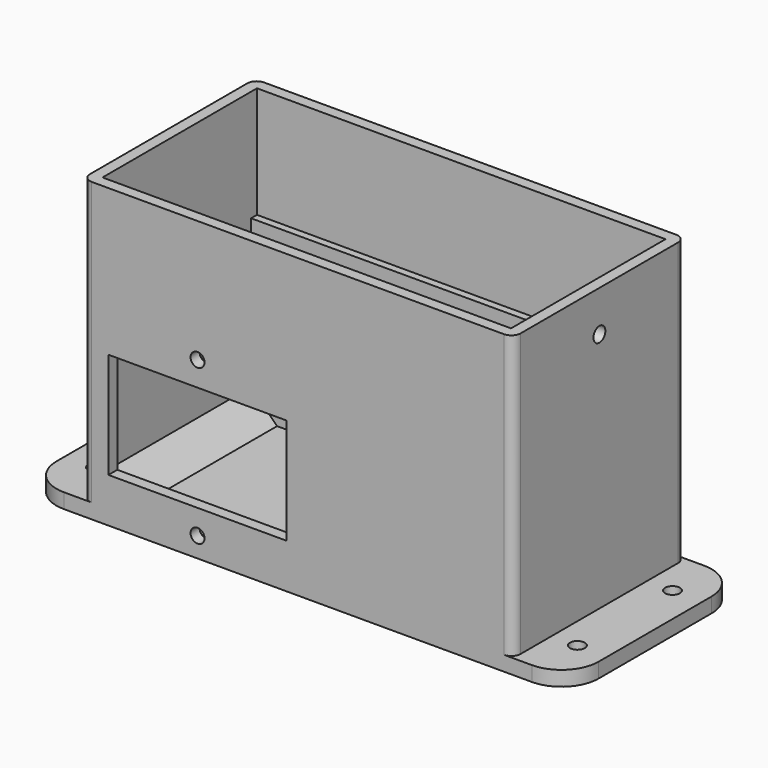
from build123d import *

# Parameters (mm, degrees)
F0_W      = 116
F0_H      = 58
F1_DEPTH  = 80
F2_T      = -3
F4_DEPTH  = 47
F5_R      = 2
F6_DEPTH  = 3.001
F7_W      = 58
F7_H      = 4
F8_DEPTH  = 15
F9_R      = 10
F10_R     = 2
F11_DEPTH = 4.001
F12_W     = 48
F12_H     = 28.5
F13_DEPTH = 5
F14_R     = 1.875
F15_DEPTH = 5
F16_W     = 25
F16_H     = 5
F17_DEPTH = 5.001
F18_R     = 2.49999
F19_R     = 2.5
F20_SIZE  = 7


# Not quite as in the source:
# - a fillet or chamfer is up to 0.001 mm smaller than in the source, because OpenCascade refuses the exact size
# - a pattern or mirror of a feature is missing from the dataset's text; its kind, count and spacing are read off the source's solid


with BuildPart() as f1:
    # F0 (on Top) → F1 (new body)
    with BuildSketch(Plane.XY):
        Rectangle(F0_W, F0_H)
    extrude(amount=F1_DEPTH)

    # F2
    f2_openings = [f1.faces().sort_by_distance(p)[0] for p in [
        (0, 0, 80),
    ]]
    offset(amount=F2_T, openings=f2_openings)

    # F3 (on face) → F4 (join)
    with BuildSketch(Plane.XY.offset(3)):
        Polygon((-55, 26), (-55, 24), (53, 24), (53, -26), (55, -26), (55, 26), align=None)
    extrude(amount=F4_DEPTH)

    # F5 (on face) → F6 (cut, through all)
    with BuildSketch(Plane(origin=(55, 0, 0), x_dir=(0, -1, 0), z_dir=(-1, 0, 0))):
        with Locations((0, 69)):
            Circle(F5_R)
    extrude(amount=-F6_DEPTH, mode=Mode.SUBTRACT)

    # F7 (on face) → F8 (join)
    with BuildSketch(Plane.YZ.offset(58)):
        with Locations((0, 2)):
            Rectangle(F7_W, F7_H)
    f8 = extrude(amount=F8_DEPTH)

    # F8_copies: F8 across plane
    add(f8.mirror(Plane(origin=(0, 0, 0), x_dir=(0, 0, -1), z_dir=(-1, 0, 0))))

    # F9
    f9_edges = [f1.edges().sort_by_distance(p)[0] for p in [
        (73, 29, 2),
        (73, -29, 2),
        (-73, -29, 2),
        (-73, 29, 2),
    ]]
    fillet(f9_edges, radius=F9_R)

    # F10 (on face) → F11 (cut, through all)
    with BuildSketch(Plane.XY.offset(4)):
        with Locations((64.8827031255, 16)):
            Circle(F10_R)
        with Locations((64.8827031255, -16)):
            Circle(F10_R)
    f11 = extrude(amount=-F11_DEPTH, mode=Mode.SUBTRACT)

    # F11_copies: F11 across plane
    add(f11.mirror(Plane(origin=(0, 0, 0), x_dir=(0, 0, -1), z_dir=(-1, 0, 0))), mode=Mode.SUBTRACT)

    # F12 (on face) → F13 (cut)
    with BuildSketch(Plane.XZ.offset(29)):
        with Locations((-27, 26.25)):
            Rectangle(F12_W, F12_H)
    extrude(amount=-F13_DEPTH, mode=Mode.SUBTRACT)

    # F14 (on face) → F15 (cut)
    with BuildSketch(Plane.XZ.offset(29)):
        with Locations((-27, 47.1)):
            Circle(F14_R)
        with Locations((-27, 5.4)):
            Circle(F14_R)
    extrude(amount=-F15_DEPTH, mode=Mode.SUBTRACT)

    # F16 (on face) → F17 (cut, through all)
    with BuildSketch(Plane.XZ.offset(-24)):
        with Locations((20.5, 10.5)):
            Rectangle(F16_W, F16_H)
    extrude(amount=-F17_DEPTH, mode=Mode.SUBTRACT)

    # F18 (radius 2.5 in the source; OpenCascade refuses exactly that, so slightly less here)
    f18_edges = [f1.edges().sort_by_distance(p)[0] for p in [
        (33, 26.5, 13),
        (8, 26.5, 13),
        (33, 26.5, 8),
        (8, 26.5, 8),
    ]]
    fillet(f18_edges, radius=F18_R)

    # F19
    f19_edges = [f1.edges().sort_by_distance(p)[0] for p in [
        (-58, -29, 42),
        (58, -29, 42),
        (58, 29, 42),
        (-58, 29, 42),
    ]]
    fillet(f19_edges, radius=F19_R)

    # F20
    f20_edges = [f1.edges().sort_by_distance(p)[0] for p in [
        (-55, -1, 3),
        (53, -1, 3),
    ]]
    chamfer(f20_edges, length=F20_SIZE)


solid = f1.part
